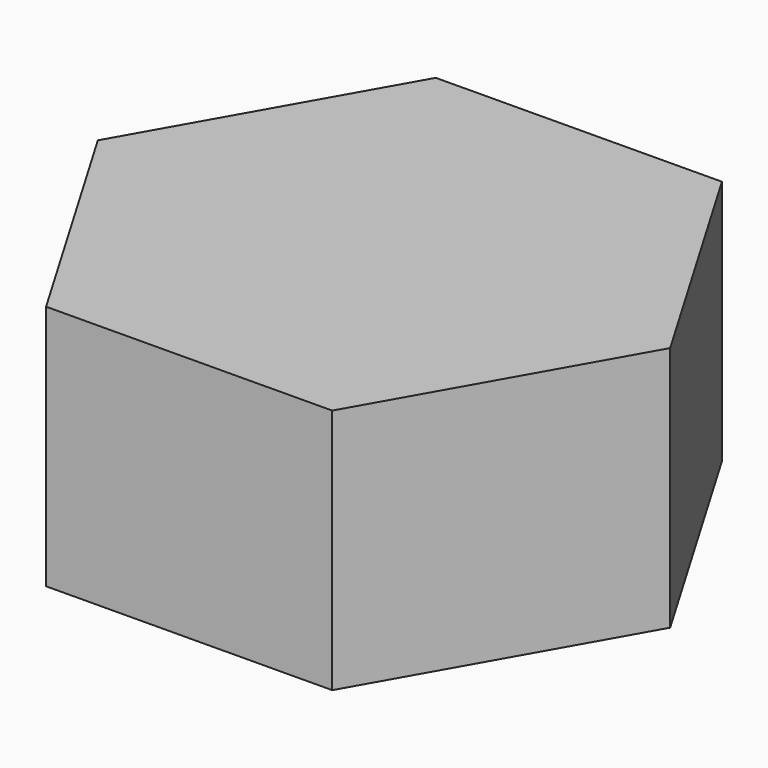
from build123d import *

# Parameters (mm, degrees)
F3_DEPTH = 4.7625
F5_DEPTH = 4.7625


# Not quite as in the source:
# - the program builds the solid bodies; features that only make, move or delete a surface that nothing else refers to are left out


with BuildPart() as f3:
    # F0 (on Top) → F3 (new body)
    with BuildSketch(Plane.XY):
        Polygon((-2.7899552341, 4.7392185946), (-5.499261314, -0.0465628108), (-2.70930608, -4.7857814054), (2.7899552341, -4.7392185946), (5.499261314, 0.0465628108), (2.70930608, 4.7857814054), align=None)
    extrude(amount=F3_DEPTH)


with BuildPart() as f5:
    # F0 (on Top) → F5 (new body)
    with BuildSketch(Plane.XY):
        Polygon((-2.7899552341, 4.7392185946), (-5.499261314, -0.0465628108), (-2.70930608, -4.7857814054), (2.7899552341, -4.7392185946), (5.499261314, 0.0465628108), (2.70930608, 4.7857814054), align=None)
    extrude(amount=F5_DEPTH)


solid = f5.part
